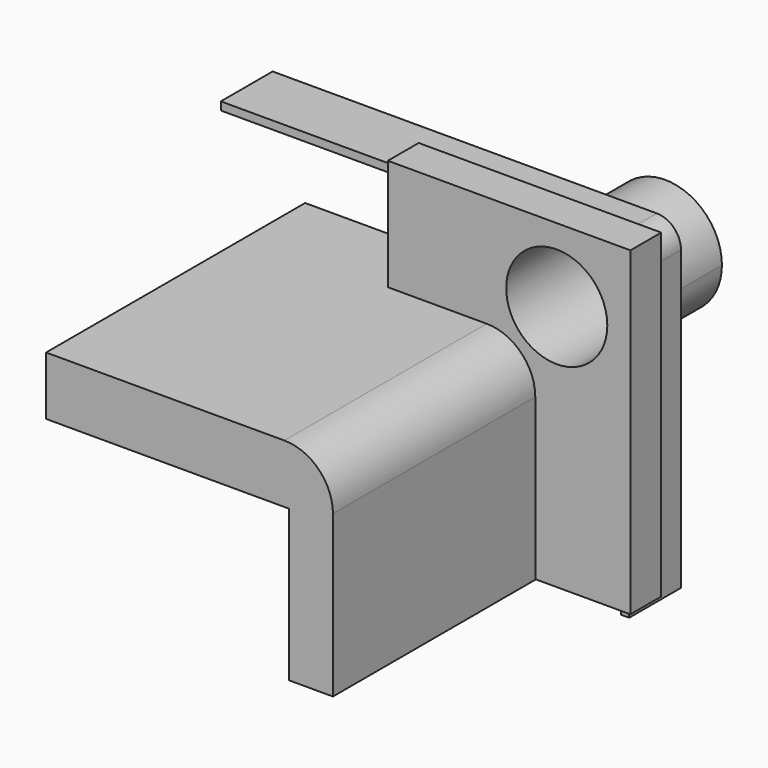
from build123d import *

# Parameters (mm, degrees)
F1_DEPTH = 127
F2_DEPTH = 25.4
F4_DEPTH = 2.4
F3_R     = 19.825
F5_DEPTH = 2.4
F6_DEPTH = 50.8
F7_DEPTH = 12.7


# Not quite as in the source:
# - a length typed as a fraction of an inch, garbled in the dataset ("3 / 203.2 mm" for 3/8 in), is restored


with BuildPart() as f1:
    # F0 (on Front) → F1 (new body)
    with BuildSketch(Plane.XZ):
        with BuildLine():
            Line((0, -82.2203159332), (0, -19.05))
            ThreePointArc((0, -19.05), (-5.5796158184, -5.5796158184), (-19.05, 0))
            Line((-19.05, 0), (-112.5172227621, 0))
            Line((-112.5172227621, 0), (-112.5172227621, -22.9479763657))
            Line((-112.5172227621, -22.9479763657), (-17.2673482448, -22.9479763657))
            Line((-17.2673482448, -22.9479763657), (-17.2673482448, -82.2203159332))
            Line((-17.2673482448, -82.2203159332), (0, -82.2203159332))
        make_face()
    extrude(amount=F1_DEPTH)


with BuildPart() as f2:
    # F0 (on Front) → F2 (new body)
    with BuildSketch(Plane.XZ):
        with BuildLine():
            Line((-125.2552419901, 41.275), (-125.2552419901, 38.1))
            Line((-125.2552419901, 38.1), (25.4, 38.1))
            ThreePointArc((25.4, 38.1), (29.8901280605, 36.2401280605), (31.75, 31.75))
            Line((31.75, 31.75), (31.75, -84.9583235416))
            Line((31.75, -84.9583235416), (34.925, -84.9583235416))
            Line((34.925, -84.9583235416), (34.925, 31.75))
            ThreePointArc((34.925, 31.75), (32.1351920908, 38.4851920908), (25.4, 41.275))
            Line((25.4, 41.275), (-125.2552419901, 41.275))
        make_face()
    extrude(amount=F2_DEPTH)


with BuildPart() as f4:
    # F3 (on face) → F4 (new body)
    with BuildSketch(Plane.XZ.offset(25.4)):
        with BuildLine():
            ThreePointArc((-8.1618525748, 0), (0.5238571529, 35.5533174442), (30.6583888685, 14.7833888685))
            ThreePointArc((30.6583888685, 14.7833888685), (20.8131820291, -3.6744372847), (0, -5.7794070793))
            Line((0, -5.7794070793), (0, -19.05))
            Line((0, -19.05), (0, -82.0128545165))
            Line((0, -82.0128545165), (31.75, -82.0128545165))
            Line((31.75, -82.0128545165), (31.75, 31.75))
            ThreePointArc((31.75, 31.75), (29.8901280605, 36.2401280605), (25.4, 38.1))
            Line((25.4, 38.1), (-57.8078702092, 38.1))
            Line((-57.8078702092, 38.1), (-57.8078702092, 0))
            Line((-57.8078702092, 0), (-19.05, 0))
            Line((-19.05, 0), (-8.1618525748, 0))
        make_face()
        with BuildLine():
            ThreePointArc((0, -5.7794070793), (-4.4102270697, -3.3547520128), (-8.1618525748, 0))
            Line((-8.1618525748, 0), (-19.05, 0))
            ThreePointArc((-19.05, 0), (-5.5796158184, -5.5796158184), (0, -19.05))
            Line((0, -19.05), (0, -5.7794070793))
        make_face()
        with BuildLine():
            Line((-57.8078702092, 41.275), (-57.8078702092, 38.1))
            Line((-57.8078702092, 38.1), (25.4, 38.1))
            ThreePointArc((25.4, 38.1), (29.8901280605, 36.2401280605), (31.75, 31.75))
            Line((31.75, 31.75), (31.75, -82.0128545165))
            Line((31.75, -82.0128545165), (34.925, -82.0128545165))
            Line((34.925, -82.0128545165), (34.925, 31.75))
            ThreePointArc((34.925, 31.75), (32.1351920908, 38.4851920908), (25.4, 41.275))
            Line((25.4, 41.275), (-57.8078702092, 41.275))
        make_face()
        with BuildLine():
            Line((-57.8078702092, 43.675), (-57.8078702092, 41.275))
            Line((-57.8078702092, 41.275), (25.4, 41.275))
            ThreePointArc((25.4, 41.275), (32.1351920908, 38.4851920908), (34.925, 31.75))
            Line((34.925, 31.75), (34.925, -82.0128545165))
            Line((34.925, -82.0128545165), (37.325, -82.0128545165))
            Line((37.325, -82.0128545165), (37.325, 43.675))
            Line((37.325, 43.675), (-57.8078702092, 43.675))
        make_face()
    extrude(amount=F4_DEPTH)

    # F3 (on face) → F5 (join, through all)
    with BuildSketch(Plane.XZ.offset(25.4)):
        with BuildLine():
            ThreePointArc((0, -5.7794070793), (20.8131820291, -3.6744372847), (30.6583888685, 14.7833888685))
            ThreePointArc((30.6583888685, 14.7833888685), (0.5238571529, 35.5533174442), (-8.1618525748, 0))
            ThreePointArc((-8.1618525748, 0), (-4.4102270697, -3.3547520128), (0, -5.7794070793))
        make_face()
        with Locations((8.4333888685, 14.7833888685)):
            Circle(F3_R, mode=Mode.SUBTRACT)
    extrude(amount=F5_DEPTH)

    # F3 (on face) → F6 (join)
    with BuildSketch(Plane.XZ.offset(25.4)):
        with BuildLine():
            ThreePointArc((0, -5.7794070793), (20.8131820291, -3.6744372847), (30.6583888685, 14.7833888685))
            ThreePointArc((30.6583888685, 14.7833888685), (0.5238571529, 35.5533174442), (-8.1618525748, 0))
            ThreePointArc((-8.1618525748, 0), (-4.4102270697, -3.3547520128), (0, -5.7794070793))
        make_face()
        with Locations((8.4333888685, 14.7833888685)):
            Circle(F3_R, mode=Mode.SUBTRACT)
    extrude(amount=-F6_DEPTH)

    # F3 (on face) → F7 (join)
    with BuildSketch(Plane.XZ.offset(25.4)):
        with BuildLine():
            Line((-57.8078702092, 43.675), (-57.8078702092, 41.275))
            Line((-57.8078702092, 41.275), (25.4, 41.275))
            ThreePointArc((25.4, 41.275), (32.1351920908, 38.4851920908), (34.925, 31.75))
            Line((34.925, 31.75), (34.925, -82.0128545165))
            Line((34.925, -82.0128545165), (37.325, -82.0128545165))
            Line((37.325, -82.0128545165), (37.325, 43.675))
            Line((37.325, 43.675), (-57.8078702092, 43.675))
        make_face()
    extrude(amount=-F7_DEPTH)


solid = Compound([f1.part, f2.part, f4.part])
